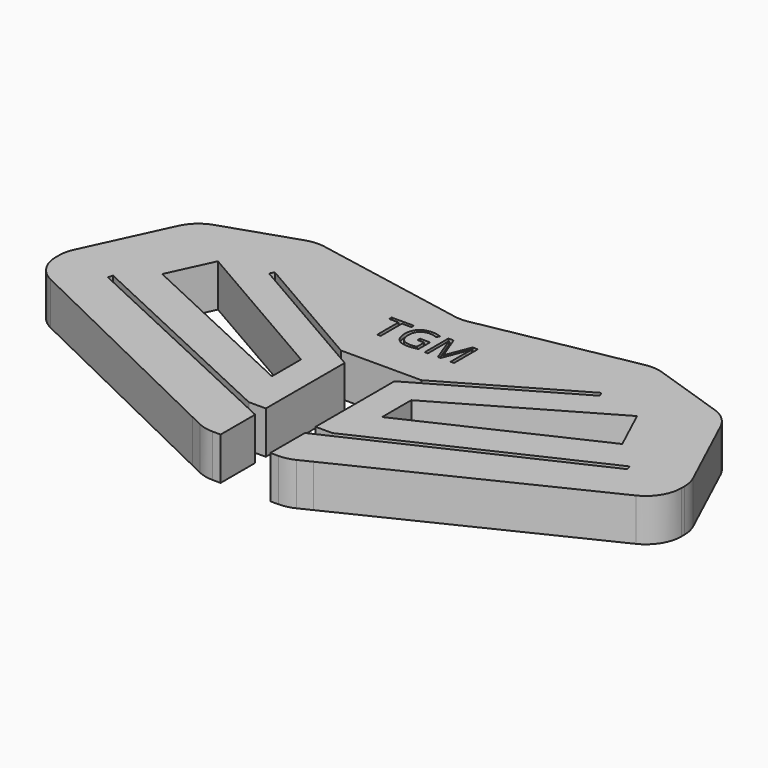
from build123d import *

# Parameters (mm, degrees)
F1_DEPTH     = 6
F2_DEPTH     = 0.2
F3_R         = 5
F5_TEXT_SIZE = 5.8398530301
F6_DEPTH     = 0.5
F7_R         = 5


# Not quite as in the source:
# - Text() gives the source's letters only with a copy of the font that has no kerning and outlines rounded to 1/6400 em; it was checked with that copy


with BuildPart() as f1:
    # F0 (on Top) → F1 (new body)
    with BuildSketch(Plane.XY):
        Polygon((-44.0399559993, 17.2425831666), (-8.5, 0), (-5.7793708718, -1.3199418145), (-3.5, -1.3199418145), (-3.5, 0), (-3.5, 4.7610669659), (-5.8936514892, 5.8772449863), (-36.5802342268, 20.1866335195), (-36.374255776, 20.8556423967), (-5.8936514892, 6.6423031926), (-3.5, 6.6423031926), (-3.5, 20.5261251722), (-5.6653383499, 21.7762838514), (-23.3031699514, 31.9594906744), (-22.9855715851, 32.584415549), (-5.6653383499, 22.5845742282), (-3.5, 22.5845742282), (0, 22.5845742282), (0, 24.010497731), (0, 25.0511443473), (0, 36.527376622), (-23.874943212, 41.0195985393), (-37.2920548999, 36.5333934459), (-44.0399559993, 21.9962090519), align=None)
        Polygon((-29.5141277367, 30.7260924555), (-7.7606518859, 18.1667173172), (-7.7606518859, 13.0297893701), (-32.3960598545, 24.5174687676), align=None, mode=Mode.SUBTRACT)
    extrude(amount=F1_DEPTH)

    # F0 (on Top) → F2 (join)
    with BuildSketch(Plane.XY):
        Polygon((-23.3031699514, 31.9594906744), (-5.6653383499, 21.7762838514), (-5.6653383499, 22.5845742282), (-22.9855715851, 32.584415549), align=None)
        Polygon((-36.5802342268, 20.1866335195), (-5.8936514892, 5.8772449863), (-5.8936514892, 6.6423031926), (-36.374255776, 20.8556423967), align=None)
    extrude(amount=F2_DEPTH)

    # F3
    f3_edges = [f1.edges().sort_by_distance(p)[0] for p in [
        (-44.039956, 17.242583, 3),
        (-44.039956, 21.996209, 3),
        (-37.292055, 36.533393, 3),
        (-23.874943, 41.019599, 3),
        (-5.779371, -1.319942, 3),
    ]]
    fillet(f3_edges, radius=F3_R)

    # F4: F1 across plane


with BuildPart() as f1_1:
    add(f1.part)
    add(f1.part.mirror(Plane.YZ))

    # F5 (on face) → F6 (cut)
    with BuildSketch(Plane.XY.offset(6)):
        with Locations((-6.2814919155, 28.0272886157)):
            Text('TGM', F5_TEXT_SIZE, font='Open Sans', text_align=(TextAlign.LEFT, TextAlign.BOTTOM))
    extrude(amount=-F6_DEPTH, mode=Mode.SUBTRACT)

    # F7
    f7_edges = [f1_1.edges().sort_by_distance(p)[0] for p in [
        (0, 36.527377, 3),
    ]]
    fillet(f7_edges, radius=F7_R)


solid = f1_1.part
